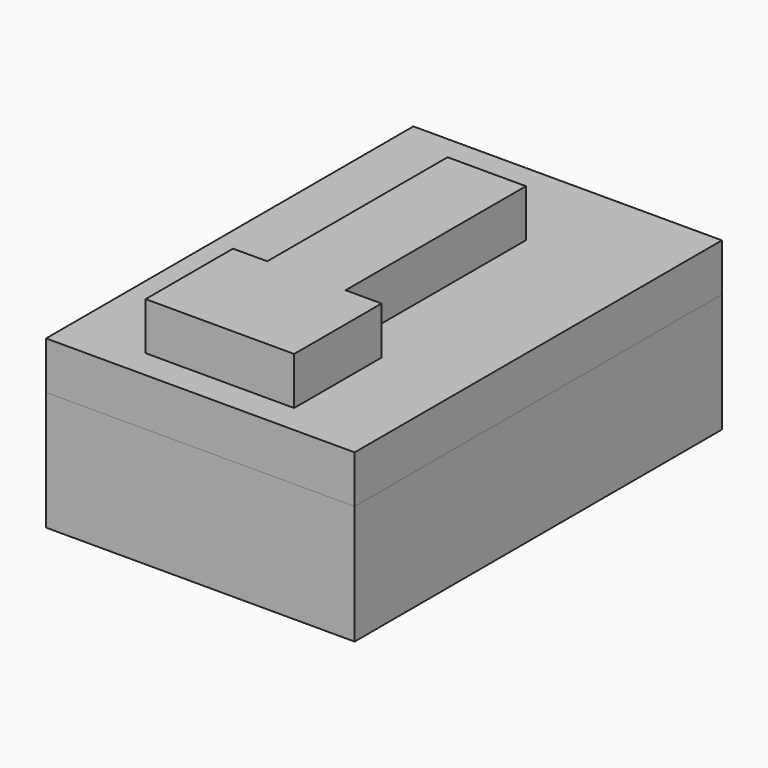
from build123d import *

# Parameters (mm, degrees)
F0_W     = 16.462284606
F0_H     = 24.4974466041
F1_DEPTH = 6.35
F2_W     = 16.462284606
F2_H     = 24.4974466041
F3_DEPTH = 2.54
F4_W     = 4.1798030725
F4_H     = 1.4798403718
F5_DEPTH = 2.54
F6_W     = 4.1798030725
F6_H     = 12.0247541927
F6_H_2   = 5.8034774847
F7_DEPTH = 2.54


# Not quite as in the source:
# - a feature names something its author has since deleted; it is built from what else it names


with BuildPart() as f1:
    # F0 (on Top) → F1 (new body)
    with BuildSketch(Plane.XY):
        with Locations((0.2442786936, 0.227171462)):
            Rectangle(F0_W, F0_H)
    extrude(amount=F1_DEPTH)


with BuildPart() as f3:
    # F2 (on face) → F3 (new body)
    with BuildSketch(Plane.XY.offset(6.35)):
        with Locations((0.2442786936, 0.227171462)):
            Rectangle(F2_W, F2_H)
    extrude(amount=F3_DEPTH)

    # F4 (on face) → F5 (cut)
    with BuildSketch(Plane.XY.offset(8.89)):
        with Locations((0.0016469858, 6.6424182151)):
            Rectangle(F4_W, F4_H)
    extrude(amount=-F5_DEPTH, mode=Mode.SUBTRACT)


with BuildPart() as f7:
    # F6 (on face) → F7 (new body)
    with BuildSketch(Plane.XY.offset(8.89)):
        with Locations((0.0016469858, 1.3699613046)):
            Rectangle(F6_W, F6_H)
        with Locations((0.0016469858, -7.5441545341)):
            Rectangle(F6_W, F6_H_2)
        Polygon((-2.0882545505, -10.4458932765), (-2.0882545505, -4.6424157917), (-3.9152200043, -4.6424157917), (-3.9152200043, -10.4728732258), (4.009673401, -10.4728732258), (4.009673401, -4.6424157917), (2.091548522, -4.6424157917), (2.091548522, -10.4458932765), align=None)
    extrude(amount=F7_DEPTH)


solid = Compound([f1.part, f3.part, f7.part])
